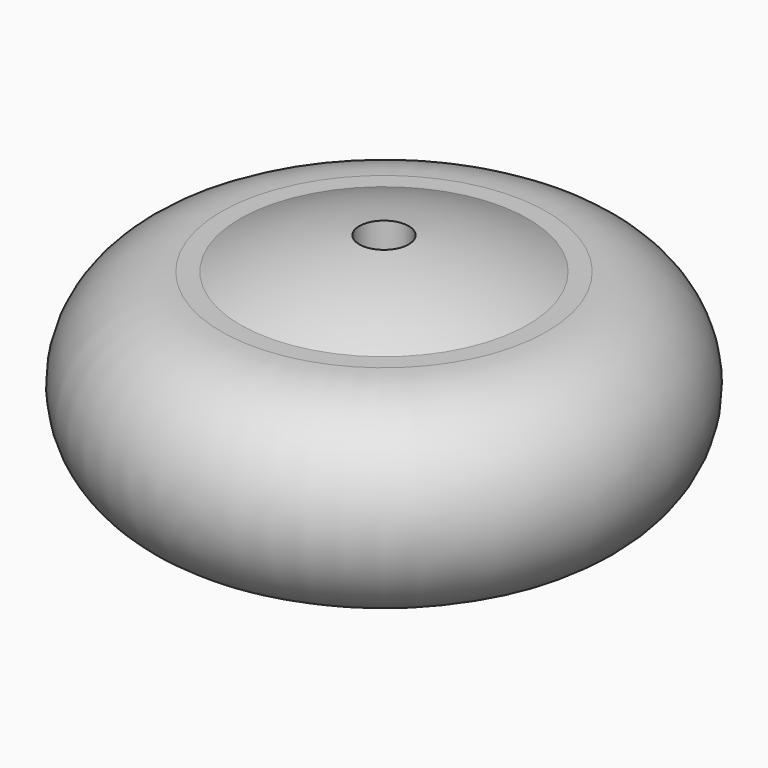
from build123d import *

# Parameters (mm, degrees)
F2_R          = 1.5
F3_DEPTH      = 7.9928655241
F3_DEPTH_BACK = 7.9998012227


with BuildPart() as f1:
    # F0 (on Front) → F1 (revolve)
    with BuildSketch(Plane.XZ):
        with BuildLine():
            Line((-9.6344217221, -5.9888523544), (-8.7234286139, -5.9891373512))
            ThreePointArc((-8.7234286139, -5.9891373512), (-4.4751851056, -7.4847544396), (0, -7.9918655241))
            Line((0, -7.9918655241), (0, 7.9988012227))
            ThreePointArc((0, 7.9988012227), (-4.4725853427, 7.4922868103), (-8.7186277917, 5.9983992579))
            Line((-8.7186277917, 5.9983992579), (-9.8591554132, 5.9983466724))
            ThreePointArc((-9.8591554132, 5.9983466724), (-15.9945732144, 0.2551312938), (-10.3693253336, -5.9886224458))
            Line((-10.3693253336, -5.9886224458), (-9.6344217221, -5.9888523544))
        make_face()
        with BuildLine():
            ThreePointArc((-10.3693253336, -5.9886224458), (-10.0018770511, -5.9999997064), (-9.6344217221, -5.9888523544))
            Line((-9.6344217221, -5.9888523544), (-10.3693253336, -5.9886224458))
        make_face()
    revolve(axis=Axis((0, 0, 0.0034678493), (0, 0, -1)))

    # F2 (on Top) → F3 (cut, two sides)
    with BuildSketch(Plane.XY) as f3_sk:
        Circle(F2_R)
    extrude(amount=-F3_DEPTH, mode=Mode.SUBTRACT)
    extrude(f3_sk.sketch, amount=F3_DEPTH_BACK, mode=Mode.SUBTRACT)


solid = f1.part
